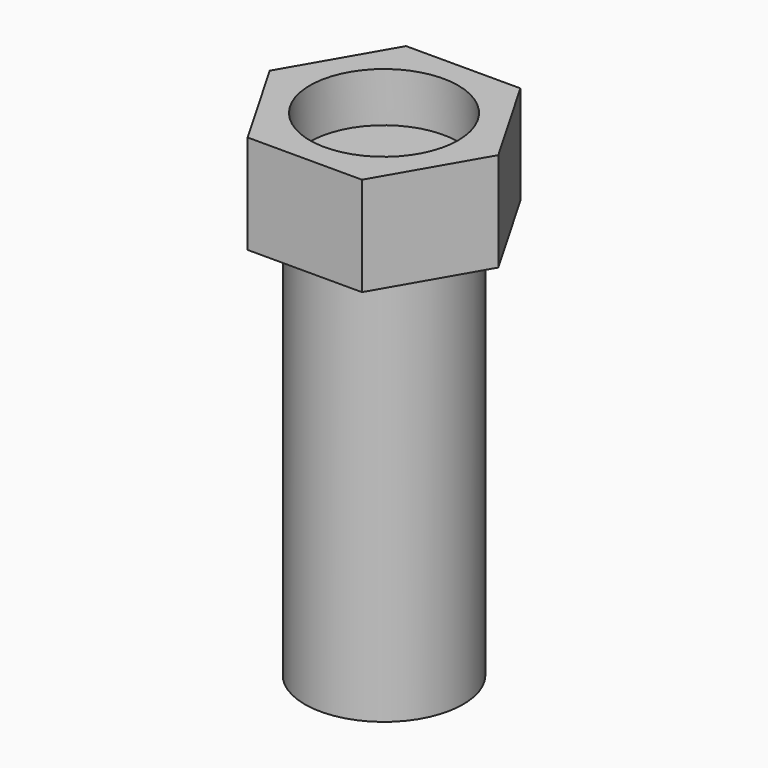
from build123d import *

# Parameters (mm, degrees)
F0_W     = 0.4
F0_H     = 2
F2_R     = 0.4
F3_DEPTH = 0.5
F4_R     = 0.375
F5_DEPTH = 0.25


with BuildPart() as f1:
    # F0 (on Front) → F1 (revolve)
    with BuildSketch(Plane.XZ):
        with Locations((-0.2, 1)):
            Rectangle(F0_W, F0_H)
    revolve(axis=Axis((0, 0, 1), (0, 0, 1)))

    # F2 (on face) → F3 (join)
    with BuildSketch(Plane.XY.offset(2)):
        Polygon((0.2886751346, 0.5), (-0.2886751346, 0.5), (-0.5773502692, 0), (-0.2886751346, -0.5), (0.2886751346, -0.5), (0.5773502692, 0), align=None)
        Circle(F2_R, mode=Mode.SUBTRACT)
        Circle(F2_R)
    extrude(amount=F3_DEPTH)

    # F4 (on face) → F5 (cut)
    with BuildSketch(Plane.XY.offset(2.5)):
        Circle(F4_R)
    extrude(amount=-F5_DEPTH, mode=Mode.SUBTRACT)


solid = f1.part
